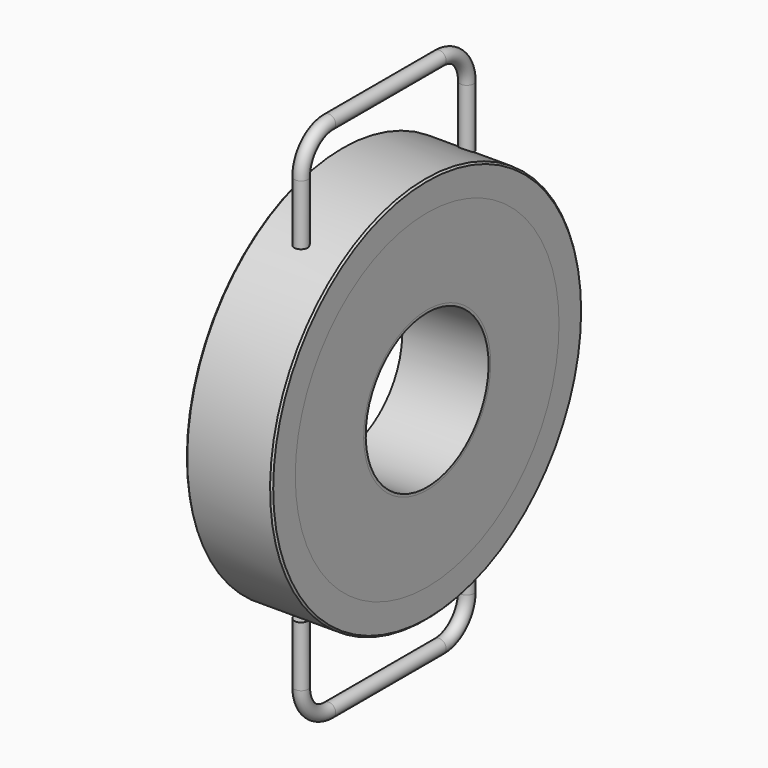
from build123d import *

# Parameters (mm, degrees)
F0_W     = 50
F0_H     = 1.5
F2_W     = 50
F2_H     = 49.5
F3_W     = 50
F3_H     = 17
F8_R     = 4
F10_SIZE = 1


# Not quite as in the source:
# - a pattern or mirror of a feature is missing from the dataset's text; its kind, count and spacing are read off the source's solid


with BuildPart() as f1:
    # F0 (on Front) → F1 (revolve)
    with BuildSketch(Plane.XZ):
        with Locations((0, 45.25)):
            Rectangle(F0_W, F0_H)
    revolve(axis=Axis((-0.9286299391, 0, 0), (1, 0, 0)))


with BuildPart() as f4:
    # F2 (on Front) → F4 (revolve)
    with BuildSketch(Plane.XZ):
        with Locations((0, 70.75)):
            Rectangle(F2_W, F2_H)
    revolve(axis=Axis((5.5879e-06, 0, 0), (1, 0, 0)))


with BuildPart() as f5:
    # F3 (on Front) → F5 (revolve)
    with BuildSketch(Plane.XZ):
        with Locations((0, 104)):
            Rectangle(F3_W, F3_H)
    revolve(axis=Axis((-0.9286299391, 0, 0), (1, 0, 0)))

    # F10
    f10_edges = [f5.edges().sort_by_distance(p)[0] for p in [
        (25, 0, -112.5),
        (-25, 0, -112.5),
    ]]
    chamfer(f10_edges, length=F10_SIZE)


with BuildPart() as f9:
    # F9: sweep along a path in F6
    with BuildLine(Plane.YZ) as f9_path:
        Line((60, 95.1643315534), (60, 130))
        ThreePointArc((60, 130), (54.1421356237, 144.1421356237), (40, 150))
        Line((40, 150), (-40, 150))
        ThreePointArc((-40, 150), (-54.1421356237, 144.1421356237), (-60, 130))
        Line((-60, 130), (-60, 95.1643315534))
    # F8 (on plane+point) → F9 (sweep)
    with BuildSketch(Plane.XY.offset(95.1643315534)):
        with Locations((0, 60)):
            Circle(F8_R)
    sweep(path=f9_path.line)


with BuildPart() as f9_copies_1:
    # F9_copies: instance of F9
    add(f9.part.mirror(Plane(origin=(0, 0, 0), x_dir=(-1, 0, 0), z_dir=(0, 0, -1))))


solid = Compound([f1.part, f4.part, f5.part, f9.part, f9_copies_1.part])
